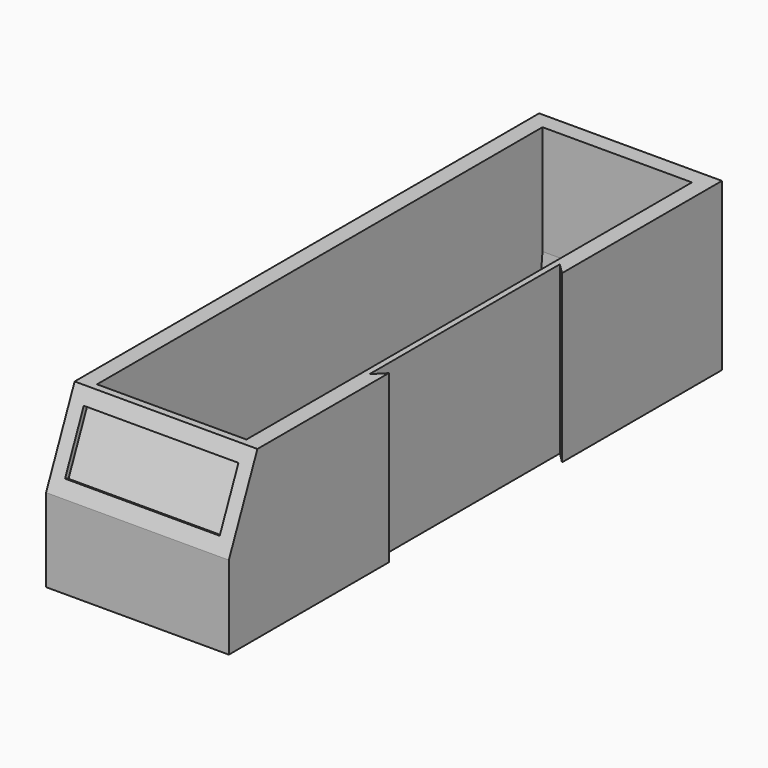
from build123d import *

# Parameters (mm, degrees)
F0_W     = 38.4
F0_H     = 129.5
F0_W_2   = 31.4
F0_H_2   = 111
F1_DEPTH = 2
F2_DEPTH = 35
F3_SIZE2 = 17.5
F3_SIZE  = 7.5
F4_SIZE2 = 32.99999
F4_SIZE  = 5.99999
F6_DEPTH = 35.001
F7_W     = 32.5
F7_H     = 12.5
F8_DEPTH = 1
F9_SIZE2 = 10
F9_SIZE  = 1


# Not quite as in the source:
# - a fillet or chamfer is up to 0.001 mm smaller than in the source, because OpenCascade refuses the exact size


with BuildPart() as f1:
    # F0 (on Top) → F1 (new body)
    with BuildSketch(Plane.XY):
        with Locations((0, -5.75)):
            Rectangle(F0_W, F0_H)
        Rectangle(F0_W_2, F0_H_2, mode=Mode.SUBTRACT)
        Rectangle(F0_W_2, F0_H_2)
    extrude(amount=F1_DEPTH)

    # F0 (on Top) → F2 (join)
    with BuildSketch(Plane.XY):
        with Locations((0, -5.75)):
            Rectangle(F0_W, F0_H)
        Rectangle(F0_W_2, F0_H_2, mode=Mode.SUBTRACT)
    extrude(amount=F2_DEPTH)

    # F3
    f3_edges = [f1.edges().sort_by_distance(p)[0] for p in [
        (0, -70.5, 35),
    ]]
    f3_side = f1.faces().sort_by_distance((0, -69.149266, 35))[0]
    chamfer(f3_edges, length=F3_SIZE, length2=F3_SIZE2, reference=f3_side)

    # F4 (size 6 and 33 in the source; OpenCascade refuses exactly that, so slightly less here)
    f4_edges = [f1.edges().sort_by_distance(p)[0] for p in [
        (0, -55.5, 35),
    ]]
    f4_side = f1.faces().sort_by_distance((17.920994, -2, 35))[0]
    chamfer(f4_edges, length=F4_SIZE, length2=F4_SIZE2, reference=f4_side)

    # F5 (on face) → F6 (cut, through all)
    with BuildSketch(Plane.XY.offset(35)):
        Polygon((19.2, -28.5), (19.2, 17), (16.95, 19.25), (16.95, -30.75), align=None)
    extrude(amount=-F6_DEPTH, mode=Mode.SUBTRACT)

    # F7 (on face) → F8 (cut)
    with BuildSketch(Plane(origin=(0, -65.8965517241, 28.2413793103), x_dir=(1, 0, 0), z_dir=(0, -0.91914503, 0.3939192986))):
        with Locations((0, -2.1665561422)):
            Rectangle(F7_W, F7_H)
    extrude(amount=-F8_DEPTH, mode=Mode.SUBTRACT)

    # F9
    f9_edges = [f1.edges().sort_by_distance(p)[0] for p in [
        (0, 55.5, 2),
    ]]
    f9_side = f1.faces().sort_by_distance((0, 0, 2))[0]
    chamfer(f9_edges, length=F9_SIZE, length2=F9_SIZE2, reference=f9_side)


solid = f1.part
